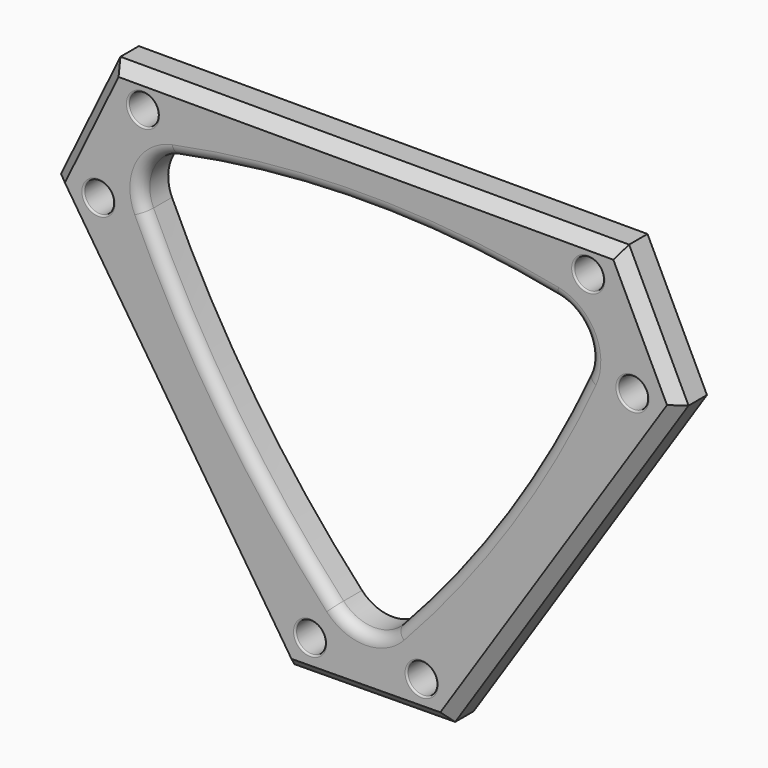
from build123d import *

# Parameters (mm, degrees)
F0_R     = 4.445
F1_DEPTH = 10.16
F2_SIZE  = 3.302
F3_R     = 3.302
F4_R     = 0.508


# Not quite as in the source:
# - ends of sketch curves that miss each other by under 0.0002 mm in the source are joined


with BuildPart() as f1:
    # F0 (on Front) → F1 (new body)
    with BuildSketch(Plane.XZ):
        Polygon((76.0178938508, 66.0481899977), (-75.6828660357, 66.0481899977), (-93.4033319354, 29.5351882561), (-23.8196160644, -76.5768140554), (24.1510938508, -76.1446207762), (93.7470938508, 29.5351882561), align=None)
        with Locations((-16.4702718891, -65.8985787277)):
            Circle(F0_R, mode=Mode.SUBTRACT)
        with Locations((16.7914066574, -65.8985787277)):
            Circle(F0_R, mode=Mode.SUBTRACT)
        with Locations((-79.6014981537, 29.1146653051)):
            Circle(F0_R, mode=Mode.SUBTRACT)
        with BuildLine():
            ThreePointArc((-56.9494813246, 46.9299354111), (-0.0054737788, 52.6137538254), (56.9385136023, 46.9297333914))
            ThreePointArc((56.9385136023, 46.9297333914), (65.5708398339, 40.3737851527), (65.7892758616, 29.5363607275))
            ThreePointArc((65.7892758616, 29.5363607275), (40.8299827062, -15.0982028275), (9.1209118413, -55.2198356451))
            ThreePointArc((9.1209118413, -55.2198356451), (0.0001026866, -59.1978132725), (-9.1209291224, -55.2203447077))
            ThreePointArc((-9.1209291224, -55.2203447077), (-40.8344645229, -15.0989921518), (-65.7996619894, 29.5351893503))
            ThreePointArc((-65.7996619894, 29.5351893503), (-65.5821849152, 40.3733311732), (-56.9494813246, 46.9299354111))
        make_face(mode=Mode.SUBTRACT)
        with Locations((-66.3161736801, 56.4890627044)):
            Circle(F0_R, mode=Mode.SUBTRACT)
        with Locations((79.6604069033, 29.5357785845)):
            Circle(F0_R, mode=Mode.SUBTRACT)
        with Locations((66.4782037265, 56.4889616946)):
            Circle(F0_R, mode=Mode.SUBTRACT)
    extrude(amount=F1_DEPTH)

    # F2
    f2_edges = [f1.edges().sort_by_distance(p)[0] for p in [
        (-84.543099, -10.16, 47.791689),
        (0.167514, -10.16, 66.04819),
        (0.165739, -10.16, -76.360717),
        (-58.611474, -10.16, -23.520813),
        (58.949094, -10.16, -23.304716),
        (84.882494, -10.16, 47.791689),
    ]]
    chamfer(f2_edges, length=F2_SIZE)

    # F3
    f3_edges = [f1.edges().sort_by_distance(p)[0] for p in [
        (-0.005474, -10.16, 52.613754),
    ]]
    fillet(f3_edges, radius=F3_R)

    # F4
    f4_edges = [f1.edges().sort_by_distance(p)[0] for p in [
        (-84.046498, -10.16, 29.114665),
        (-70.761174, -10.16, 56.489063),
        (62.033204, -10.16, 56.488962),
        (75.215407, -10.16, 29.535779),
        (-20.915272, -10.16, -65.898579),
        (12.346407, -10.16, -65.898579),
    ]]
    fillet(f4_edges, radius=F4_R)


solid = f1.part
